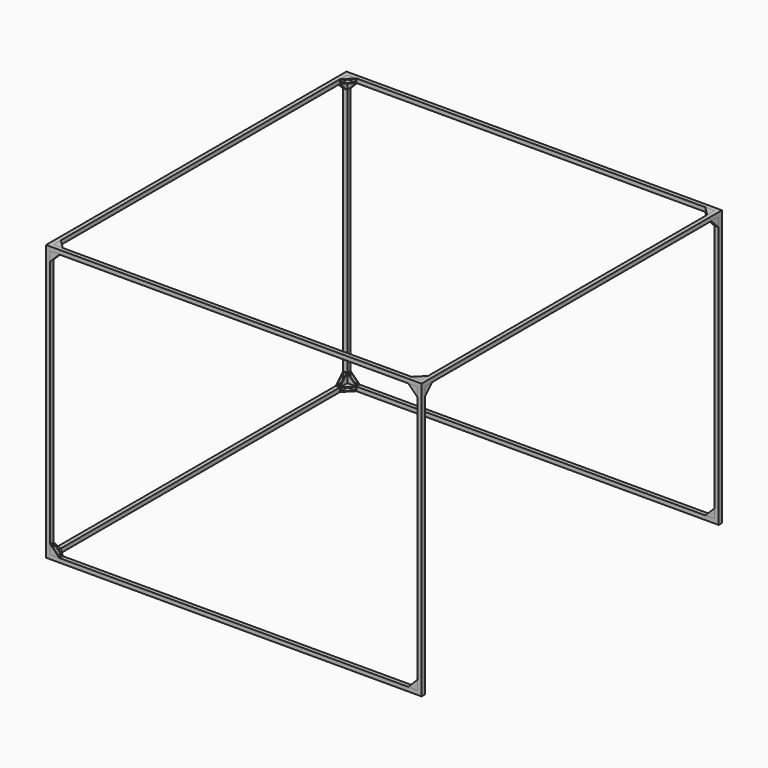
from build123d import *

# Parameters (mm, degrees)
F0_W      = 4000
F0_H      = 45
F1_DEPTH  = 45
F4_W      = 45
F4_H      = 4000
F5_DEPTH  = 45
F6_W      = 4000
F6_H      = 45
F7_DEPTH  = 45
F9_DEPTH  = 45
F14_DEPTH = 45
F18_DEPTH = 45
F23_T     = -5
F23_2_T   = -5
F23_3_T   = -5
F23_4_T   = -5
F23_5_T   = -5
F23_6_T   = -5
F23_7_T   = -5
F23_8_T   = -5
F23_9_T   = -5
F23_10_T  = -5
F23_11_T  = -5
F23_12_T  = -5
F23_13_T  = -5
F23_14_T  = -5
F23_15_T  = -5
F23_16_T  = -5
F23_17_T  = -5
F23_18_T  = -5
F23_19_T  = -5
F23_20_T  = -5
F25_DEPTH = 25


with BuildPart() as f1:
    # F0 (on Front) → F1 (new body)
    with BuildSketch(Plane.XZ):
        Polygon((-169.6427954237, 1461.3917125762), (-214.6427954237, 1461.3917125762), (-214.6427954237, -1538.6082874238), (-169.6427954237, -1538.6082874238), (-169.6427954237, -1493.6082874238), (-169.6427954237, 1416.3917125762), align=None)
        Polygon((3875.3572045763, 1461.3917125762), (3830.3572045763, 1461.3917125762), (3830.3572045763, 1416.3917125762), (3830.3572045763, -1493.6082874238), (3830.3572045763, -1538.6082874238), (3875.3572045763, -1538.6082874238), align=None)
        with Locations((1830.3572045763, 1438.8917125762)):
            Rectangle(F0_W, F0_H)
        with Locations((1830.3572045763, -1516.1082874238)):
            Rectangle(F0_W, F0_H)
    extrude(amount=F1_DEPTH)


with BuildPart() as f3_1:
    # F3: instance of F1
    add(f1.part.mirror(Plane(origin=(1830.3572045763, -2045, -38.6082874238), x_dir=(1, 0, 0), z_dir=(0, -1, 0))))


with BuildPart() as f1_1:
    add(f1.part)

    add(f3_1.part)  # F5 merges F3_1
    # F4 (on face) → F5 (join)
    with BuildSketch(Plane.XY.offset(1461.3917125762)):
        with Locations((3852.8572045763, -2045)):
            Rectangle(F4_W, F4_H)
        with Locations((-192.1427954237, -2045)):
            Rectangle(F4_W, F4_H)
    extrude(amount=-F5_DEPTH)

    # F6 (on face) → F7 (join)
    with BuildSketch(Plane(origin=(-214.6427954237, 0, 0), x_dir=(0, -1, 0), z_dir=(-1, 0, 0))):
        with Locations((2045, -1516.1082874238)):
            Rectangle(F6_W, F6_H)
    extrude(amount=-F7_DEPTH)


with BuildPart() as f9:
    # F8 (on face) → F9 (new body)
    with BuildSketch(Plane.YZ.offset(3875.3572045763)):
        Polygon((-4045, 1316.3917125762), (-3945, 1416.3917125762), (-4045, 1416.3917125762), align=None)
    extrude(amount=-F9_DEPTH)


with BuildPart() as f10_1:
    # F10: instance of F9
    add(f9.part.mirror(Plane(origin=(1830.3572045763, -2045, -38.6082874238), x_dir=(1, 0, 0), z_dir=(0, -1, 0))))


with BuildPart() as f12_1:
    # F12: instance of F9
    add(f9.part.mirror(Plane(origin=(1830.3572045763, -2045, 1438.8917125762), x_dir=(0, -1, 0), z_dir=(-1, 0, 0))))


with BuildPart() as f12_2:
    # F12: instance of F10_1
    add(f10_1.part.mirror(Plane(origin=(1830.3572045763, -2045, 1438.8917125762), x_dir=(0, -1, 0), z_dir=(-1, 0, 0))))


with BuildPart() as f14:
    # F13 (on face) → F14 (new body)
    with BuildSketch(Plane(origin=(0, 0, 0), x_dir=(-1, 0, 0), z_dir=(0, 1, 0))):
        Polygon((-3730.3572045763, 1416.3917125762), (-3830.3572045763, 1416.3917125762), (-3830.3572045763, 1316.3917125762), align=None)
    extrude(amount=-F14_DEPTH)


with BuildPart() as f15_1:
    # F15: instance of F14
    add(f14.part.mirror(Plane(origin=(1830.3572045763, -2045, 1438.8917125762), x_dir=(0, -1, 0), z_dir=(-1, 0, 0))))


with BuildPart() as f16_1:
    # F16: instance of F14
    add(f14.part.mirror(Plane(origin=(1830.3572045763, -2045, -38.6082874238), x_dir=(1, 0, 0), z_dir=(0, -1, 0))))


with BuildPart() as f16_2:
    # F16: instance of F15_1
    add(f15_1.part.mirror(Plane(origin=(1830.3572045763, -2045, -38.6082874238), x_dir=(1, 0, 0), z_dir=(0, -1, 0))))


with BuildPart() as f18:
    # F17 (on face) → F18 (new body)
    with BuildSketch(Plane.XY.offset(1461.3917125762)):
        Polygon((-169.6427954237, -3945), (-169.6427954237, -4045), (-69.6427954237, -4045), align=None)
    extrude(amount=-F18_DEPTH)


with BuildPart() as f19_1:
    # F19: instance of F18
    add(f18.part.mirror(Plane(origin=(1830.3572045763, -2045, 1438.8917125762), x_dir=(0, -1, 0), z_dir=(-1, 0, 0))))


with BuildPart() as f20_1:
    # F20: instance of F18
    add(f18.part.mirror(Plane(origin=(1830.3572045763, -2045, -38.6082874238), x_dir=(1, 0, 0), z_dir=(0, -1, 0))))


with BuildPart() as f20_2:
    # F20: instance of F19_1
    add(f19_1.part.mirror(Plane(origin=(1830.3572045763, -2045, -38.6082874238), x_dir=(1, 0, 0), z_dir=(0, -1, 0))))

    # F23#7
    f23_7_openings = [f20_2.faces().sort_by_distance(p)[0] for p in [
        (3780.357205, -95, 1438.891713),
    ]]
    offset(amount=F23_7_T, openings=f23_7_openings)


with BuildPart() as f22_1:
    # F22: instance of F14
    add(f14.part.mirror(Plane(origin=(1830.3572045763, -22.5, -38.6082874238), x_dir=(1, 0, 0), z_dir=(0, 0, -1))))

    # F23#16
    f23_16_openings = [f22_1.faces().sort_by_distance(p)[0] for p in [
        (3780.357205, -22.5, -1443.608287),
    ]]
    offset(amount=F23_16_T, openings=f23_16_openings)


with BuildPart() as f22_2:
    # F22: instance of F15_1
    add(f15_1.part.mirror(Plane(origin=(1830.3572045763, -22.5, -38.6082874238), x_dir=(1, 0, 0), z_dir=(0, 0, -1))))

    # F23#2
    f23_2_openings = [f22_2.faces().sort_by_distance(p)[0] for p in [
        (-119.642795, -22.5, -1443.608287),
    ]]
    offset(amount=F23_2_T, openings=f23_2_openings)


with BuildPart() as f22_3:
    # F22: instance of F16_1
    add(f16_1.part.mirror(Plane(origin=(1830.3572045763, -22.5, -38.6082874238), x_dir=(1, 0, 0), z_dir=(0, 0, -1))))

    # F23#17
    f23_17_openings = [f22_3.faces().sort_by_distance(p)[0] for p in [
        (3780.357205, -4067.5, -1443.608287),
    ]]
    offset(amount=F23_17_T, openings=f23_17_openings)


with BuildPart() as f22_4:
    # F22: instance of F16_2
    add(f16_2.part.mirror(Plane(origin=(1830.3572045763, -22.5, -38.6082874238), x_dir=(1, 0, 0), z_dir=(0, 0, -1))))

    # F23#18
    f23_18_openings = [f22_4.faces().sort_by_distance(p)[0] for p in [
        (-119.642795, -4067.5, -1443.608287),
    ]]
    offset(amount=F23_18_T, openings=f23_18_openings)


with BuildPart() as f22_5:
    # F22: instance of F12_2
    add(f12_2.part.mirror(Plane(origin=(1830.3572045763, -22.5, -38.6082874238), x_dir=(1, 0, 0), z_dir=(0, 0, -1))))

    # F23
    f23_openings = [f22_5.faces().sort_by_distance(p)[0] for p in [
        (-192.142795, -95, -1443.608287),
    ]]
    offset(amount=F23_T, openings=f23_openings)


with BuildPart() as f22_6:
    # F22: instance of F12_1
    add(f12_1.part.mirror(Plane(origin=(1830.3572045763, -22.5, -38.6082874238), x_dir=(1, 0, 0), z_dir=(0, 0, -1))))

    # F23#20
    f23_20_openings = [f22_6.faces().sort_by_distance(p)[0] for p in [
        (-192.142795, -3995, -1443.608287),
    ]]
    offset(amount=F23_20_T, openings=f23_20_openings)


with BuildPart() as f22_7:
    # F22: instance of F20_1
    add(f20_1.part.mirror(Plane(origin=(1830.3572045763, -22.5, -38.6082874238), x_dir=(1, 0, 0), z_dir=(0, 0, -1))))

    # F23#3
    f23_3_openings = [f22_7.faces().sort_by_distance(p)[0] for p in [
        (-119.642795, -95, -1516.108287),
    ]]
    offset(amount=F23_3_T, openings=f23_3_openings)


with BuildPart() as f22_8:
    # F22: instance of F18
    add(f18.part.mirror(Plane(origin=(1830.3572045763, -22.5, -38.6082874238), x_dir=(1, 0, 0), z_dir=(0, 0, -1))))

    # F23#19
    f23_19_openings = [f22_8.faces().sort_by_distance(p)[0] for p in [
        (-119.642795, -3995, -1516.108287),
    ]]
    offset(amount=F23_19_T, openings=f23_19_openings)


with BuildPart() as f20_1_1:
    add(f20_1.part)

    # F23#4
    f23_4_openings = [f20_1_1.faces().sort_by_distance(p)[0] for p in [
        (-119.642795, -95, 1438.891713),
    ]]
    offset(amount=F23_4_T, openings=f23_4_openings)


with BuildPart() as f12_2_1:
    add(f12_2.part)

    # F23#5
    f23_5_openings = [f12_2_1.faces().sort_by_distance(p)[0] for p in [
        (-192.142795, -95, 1366.391713),
    ]]
    offset(amount=F23_5_T, openings=f23_5_openings)


with BuildPart() as f15_1_1:
    add(f15_1.part)

    # F23#6
    f23_6_openings = [f15_1_1.faces().sort_by_distance(p)[0] for p in [
        (-119.642795, -22.5, 1366.391713),
    ]]
    offset(amount=F23_6_T, openings=f23_6_openings)


with BuildPart() as f10_1_1:
    add(f10_1.part)

    # F23#8
    f23_8_openings = [f10_1_1.faces().sort_by_distance(p)[0] for p in [
        (3852.857205, -95, 1366.391713),
    ]]
    offset(amount=F23_8_T, openings=f23_8_openings)


with BuildPart() as f14_1:
    add(f14.part)

    # F23#9
    f23_9_openings = [f14_1.faces().sort_by_distance(p)[0] for p in [
        (3780.357205, -22.5, 1366.391713),
    ]]
    offset(amount=F23_9_T, openings=f23_9_openings)


with BuildPart() as f19_1_1:
    add(f19_1.part)

    # F23#10
    f23_10_openings = [f19_1_1.faces().sort_by_distance(p)[0] for p in [
        (3780.357205, -3995, 1438.891713),
    ]]
    offset(amount=F23_10_T, openings=f23_10_openings)

    # F24 (on face) → F25 (cut)
    with BuildSketch(Plane(origin=(3825.3572045763, 0, 0), x_dir=(0, -1, 0), z_dir=(-1, 0, 0))):
        with BuildLine():
            Line((3982.8212277441, 1443.8917125762), (3977.8212277441, 1443.8917125762))
            ThreePointArc((3977.8212277441, 1443.8917125762), (3972.8212277441, 1438.8917125762), (3977.8212277441, 1433.8917125762))
            Line((3977.8212277441, 1433.8917125762), (3982.8212277441, 1433.8917125762))
            ThreePointArc((3982.8212277441, 1433.8917125762), (3987.8212277441, 1438.8917125762), (3982.8212277441, 1443.8917125762))
        make_face()
        with BuildLine():
            ThreePointArc((4007.1787722559, 1443.8917125762), (4002.1787722559, 1438.8917125762), (4007.1787722559, 1433.8917125762))
            Line((4007.1787722559, 1433.8917125762), (4012.1787722559, 1433.8917125762))
            ThreePointArc((4012.1787722559, 1433.8917125762), (4017.1787722559, 1438.8917125762), (4012.1787722559, 1443.8917125762))
            Line((4012.1787722559, 1443.8917125762), (4007.1787722559, 1443.8917125762))
        make_face()
    extrude(amount=-F25_DEPTH, mode=Mode.SUBTRACT)


with BuildPart() as f9_1:
    add(f9.part)

    # F23#11
    f23_11_openings = [f9_1.faces().sort_by_distance(p)[0] for p in [
        (3852.857205, -3995, 1366.391713),
    ]]
    offset(amount=F23_11_T, openings=f23_11_openings)


with BuildPart() as f16_1_1:
    add(f16_1.part)

    # F23#12
    f23_12_openings = [f16_1_1.faces().sort_by_distance(p)[0] for p in [
        (3780.357205, -4067.5, 1366.391713),
    ]]
    offset(amount=F23_12_T, openings=f23_12_openings)


with BuildPart() as f18_1:
    add(f18.part)

    # F23#13
    f23_13_openings = [f18_1.faces().sort_by_distance(p)[0] for p in [
        (-119.642795, -3995, 1438.891713),
    ]]
    offset(amount=F23_13_T, openings=f23_13_openings)


with BuildPart() as f16_2_1:
    add(f16_2.part)

    # F23#14
    f23_14_openings = [f16_2_1.faces().sort_by_distance(p)[0] for p in [
        (-119.642795, -4067.5, 1366.391713),
    ]]
    offset(amount=F23_14_T, openings=f23_14_openings)


with BuildPart() as f12_1_1:
    add(f12_1.part)

    # F23#15
    f23_15_openings = [f12_1_1.faces().sort_by_distance(p)[0] for p in [
        (-192.142795, -3995, 1366.391713),
    ]]
    offset(amount=F23_15_T, openings=f23_15_openings)


solid = Compound([f1_1.part, f20_2.part, f22_1.part, f22_2.part, f22_3.part, f22_4.part, f22_5.part, f22_6.part, f22_7.part, f22_8.part, f20_1_1.part, f12_2_1.part, f15_1_1.part, f10_1_1.part, f14_1.part, f19_1_1.part, f9_1.part, f16_1_1.part, f18_1.part, f16_2_1.part, f12_1_1.part])
